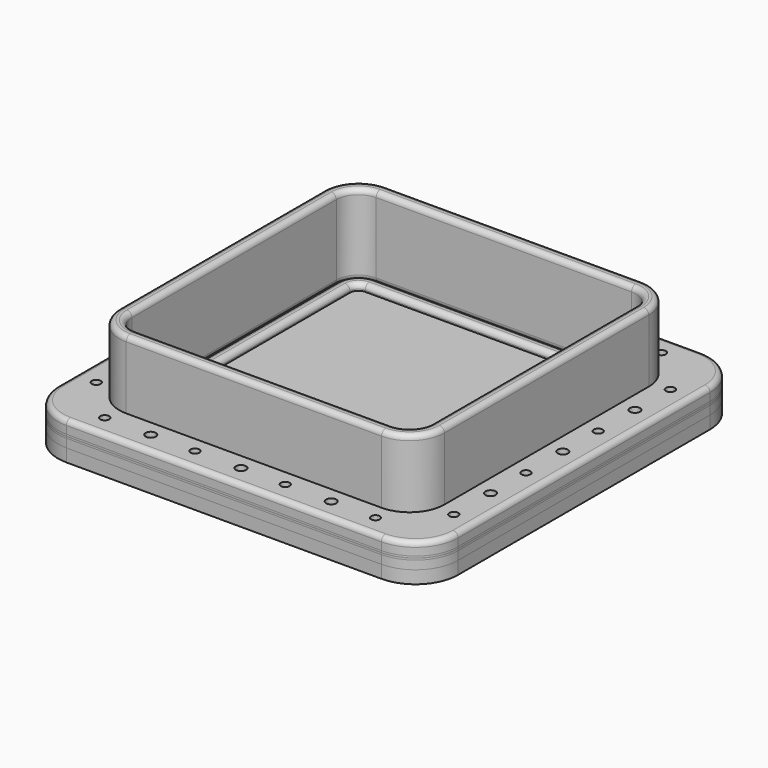
from build123d import *

# Parameters (mm, degrees)
F1_DEPTH  = 25
F2_DEPTH  = 10
F3_R      = 3
F4_DEPTH  = 7.5
F6_DEPTH  = 25
F8_DEPTH  = 40
F9_R      = 3
F10_R     = 3
F11_R     = 2.6
F13_DEPTH = 25
F14_R     = 2.6
F15_DEPTH = 1
F16_R     = 2.6
F17_DEPTH = 0.1
F18_R     = 2.6
F19_DEPTH = 1
F20_R     = 2.6
F21_DEPTH = 5
F23_DEPTH = 7.5
F25_DEPTH = 10
F26_R     = 3
F28_D     = 6
F28_2_D   = 6
F28_3_D   = 6
F28_4_D   = 6
F28_5_D   = 6
F28_6_D   = 6


# Not quite as in the source:
# - a feature names something its author has since deleted; it is built from what else it names


with BuildPart() as f1:
    # F0 (on Top) → F1 (new body)
    with BuildSketch(Plane.XY):
        with BuildLine():
            Line((-75, -87.5), (75, -87.5))
            ThreePointArc((75, -87.5), (83.8388347648, -83.8388347648), (87.5, -75))
            Line((87.5, -75), (87.5, 75))
            ThreePointArc((87.5, 75), (83.8388347648, 83.8388347648), (75, 87.5))
            Line((75, 87.5), (-75, 87.5))
            ThreePointArc((-75, 87.5), (-83.8388347648, 83.8388347648), (-87.5, 75))
            Line((-87.5, 75), (-87.5, -75))
            ThreePointArc((-87.5, -75), (-83.8388347648, -83.8388347648), (-75, -87.5))
        make_face()
        with BuildLine():
            ThreePointArc((80, -75), (78.5355339059, -78.5355339059), (75, -80))
            Line((75, -80), (-75, -80))
            ThreePointArc((-75, -80), (-78.5355339059, -78.5355339059), (-80, -75))
            Line((-80, -75), (-80, 75))
            ThreePointArc((-80, 75), (-78.5355339059, 78.5355339059), (-75, 80))
            Line((-75, 80), (75, 80))
            ThreePointArc((75, 80), (78.5355339059, 78.5355339059), (80, 75))
            Line((80, 75), (80, -75))
        make_face(mode=Mode.SUBTRACT)
    extrude(amount=F1_DEPTH)

    # F0 (on Top) → F2 (join)
    with BuildSketch(Plane.XY):
        with BuildLine():
            Line((-92.5, -117.5), (92.5, -117.5))
            ThreePointArc((92.5, -117.5), (110.1776695297, -110.1776695297), (117.5, -92.5))
            Line((117.5, -92.5), (117.5, 92.5))
            ThreePointArc((117.5, 92.5), (110.1776695297, 110.1776695297), (92.5, 117.5))
            Line((92.5, 117.5), (-92.5, 117.5))
            ThreePointArc((-92.5, 117.5), (-110.1776695297, 110.1776695297), (-117.5, 92.5))
            Line((-117.5, 92.5), (-117.5, -92.5))
            ThreePointArc((-117.5, -92.5), (-110.1776695297, -110.1776695297), (-92.5, -117.5))
        make_face()
        with BuildLine():
            ThreePointArc((87.5, -75), (83.8388347648, -83.8388347648), (75, -87.5))
            Line((75, -87.5), (-75, -87.5))
            ThreePointArc((-75, -87.5), (-83.8388347648, -83.8388347648), (-87.5, -75))
            Line((-87.5, -75), (-87.5, 75))
            ThreePointArc((-87.5, 75), (-83.8388347648, 83.8388347648), (-75, 87.5))
            Line((-75, 87.5), (75, 87.5))
            ThreePointArc((75, 87.5), (83.8388347648, 83.8388347648), (87.5, 75))
            Line((87.5, 75), (87.5, -75))
        make_face(mode=Mode.SUBTRACT)
    extrude(amount=F2_DEPTH)

    # F3
    f3_edges = [f1.edges().sort_by_distance(p)[0] for p in [
        (0, -87.5, 25),
        (83.838835, -83.838835, 25),
        (87.5, 0, 25),
        (83.838835, 83.838835, 25),
        (0, 87.5, 25),
        (-83.838835, 83.838835, 25),
        (-87.5, 0, 25),
        (-83.838835, -83.838835, 25),
        (78.535534, -78.535534, 25),
        (0, -80, 25),
        (-78.535534, -78.535534, 25),
        (-80, 0, 25),
        (-78.535534, 78.535534, 25),
        (0, 80, 25),
        (78.535534, 78.535534, 25),
        (80, 0, 25),
    ]]
    fillet(f3_edges, radius=F3_R)


with BuildPart() as f4:
    # F4 (new): a face of the model
    f4_faces = [f1.part.faces().sort_by_distance(p)[0] for p in [
        (-107.8276695297, -107.8276695297, 10),
    ]]
    extrude(f4_faces, amount=F4_DEPTH)


with BuildPart() as f6_tool:
    # F5 (on face) → F6 (new body)
    with BuildSketch(Plane.XY.offset(17.5)):
        with BuildLine():
            Line((-75, -88), (75, -88))
            ThreePointArc((75, -88), (84.1923881554, -84.1923881554), (88, -75))
            Line((88, -75), (88, 75))
            ThreePointArc((88, 75), (84.1923881554, 84.1923881554), (75, 88))
            Line((75, 88), (-75, 88))
            ThreePointArc((-75, 88), (-84.1923881554, 84.1923881554), (-88, 75))
            Line((-88, 75), (-88, -75))
            ThreePointArc((-88, -75), (-84.1923881554, -84.1923881554), (-75, -88))
        make_face()
    extrude(amount=-F6_DEPTH)


with BuildPart() as f1_1:
    add(f1.part)

    # F6: cut by f6_tool
    add(f6_tool.part, mode=Mode.SUBTRACT)


with BuildPart() as f4_1:
    add(f4.part)

    # F6: cut by f6_tool
    add(f6_tool.part, mode=Mode.SUBTRACT)

    # F7 (on face) → F8 (join)
    with BuildSketch(Plane.XY.offset(17.5)):
        with BuildLine():
            Line((-75, -95.5), (75, -95.5))
            ThreePointArc((75, -95.5), (89.4956890143, -89.4956890143), (95.5, -75))
            Line((95.5, -75), (95.5, 75))
            ThreePointArc((95.5, 75), (89.4956890143, 89.4956890143), (75, 95.5))
            Line((75, 95.5), (-75, 95.5))
            ThreePointArc((-75, 95.5), (-89.4956890143, 89.4956890143), (-95.5, 75))
            Line((-95.5, 75), (-95.5, -75))
            ThreePointArc((-95.5, -75), (-89.4956890143, -89.4956890143), (-75, -95.5))
        make_face()
        with BuildLine():
            ThreePointArc((88, -75), (84.1923881554, -84.1923881554), (75, -88))
            Line((75, -88), (-75, -88))
            ThreePointArc((-75, -88), (-84.1923881554, -84.1923881554), (-88, -75))
            Line((-88, -75), (-88, 75))
            ThreePointArc((-88, 75), (-84.1923881554, 84.1923881554), (-75, 88))
            Line((-75, 88), (75, 88))
            ThreePointArc((75, 88), (84.1923881554, 84.1923881554), (88, 75))
            Line((88, 75), (88, -75))
        make_face(mode=Mode.SUBTRACT)
    extrude(amount=F8_DEPTH)

    # F9
    f9_edges = [f4_1.edges().sort_by_distance(p)[0] for p in [
        (0, -95.5, 57.5),
        (89.495689, -89.495689, 57.5),
        (95.5, 0, 57.5),
        (89.495689, 89.495689, 57.5),
        (0, 95.5, 57.5),
        (-89.495689, 89.495689, 57.5),
        (-95.5, 0, 57.5),
        (-89.495689, -89.495689, 57.5),
        (84.192388, -84.192388, 57.5),
        (0, -88, 57.5),
        (-84.192388, -84.192388, 57.5),
        (-88, 0, 57.5),
        (-84.192388, 84.192388, 57.5),
        (0, 88, 57.5),
        (84.192388, 84.192388, 57.5),
        (88, 0, 57.5),
        (0, 117.5, 17.5),
    ]]
    fillet(f9_edges, radius=F9_R)

    # F10
    f10_edges = [f4_1.edges().sort_by_distance(p)[0] for p in [
        (0, -88, 10),
    ]]
    fillet(f10_edges, radius=F10_R)

    # F11 (on face) → F13 (cut)
    with BuildSketch(Plane(origin=(0, 0, 0), x_dir=(1, 0, 0), z_dir=(0, 0, -1))):
        with Locations((-80, 105)):
            Circle(F11_R)
        with Locations((-105, 80)):
            Circle(F11_R)
        with Locations((-80, -105)):
            Circle(F11_R)
        with Locations((-27, 105)):
            Circle(F11_R)
        with Locations((-27, -105)):
            Circle(F11_R)
        with Locations((26, 105)):
            Circle(F11_R)
        with Locations((26, -105)):
            Circle(F11_R)
        with Locations((79, 105)):
            Circle(F11_R)
        with Locations((79, -105)):
            Circle(F11_R)
        with Locations((-105, 27)):
            Circle(F11_R)
        with Locations((-105, -26)):
            Circle(F11_R)
        with Locations((-105, -79)):
            Circle(F11_R)
        with Locations((105, 80)):
            Circle(F11_R)
        with Locations((105, 27)):
            Circle(F11_R)
        with Locations((105, -26)):
            Circle(F11_R)
        with Locations((105, -79)):
            Circle(F11_R)
    extrude(amount=-F13_DEPTH, mode=Mode.SUBTRACT)

    # F28 (through all)
    with Locations(Plane(origin=(0, 0, -4.6), x_dir=(1, 0, 0), z_dir=(0, 0, -1))):
        with Locations((-105, 53), (-105, 0), (-105, -53), (-53, -105), (0, -105), (53, -105), (105, -53), (105, 0), (105, 53), (53, 105), (0, 105), (-53, 105)):
            Hole(F28_D / 2)


with BuildPart() as f15:
    # F14 (on face) → F15 (new body)
    with BuildSketch(Plane(origin=(0, 0, 10), x_dir=(1, 0, 0), z_dir=(0, 0, -1))):
        with BuildLine():
            ThreePointArc((117.5, 92.5), (110.1776695297, 110.1776695297), (92.5, 117.5))
            Line((92.5, 117.5), (-92.5, 117.5))
            ThreePointArc((-92.5, 117.5), (-110.1776695297, 110.1776695297), (-117.5, 92.5))
            Line((-117.5, 92.5), (-117.5, -92.5))
            ThreePointArc((-117.5, -92.5), (-110.1776695297, -110.1776695297), (-92.5, -117.5))
            Line((-92.5, -117.5), (92.5, -117.5))
            ThreePointArc((92.5, -117.5), (110.1776695297, -110.1776695297), (117.5, -92.5))
            Line((117.5, -92.5), (117.5, 92.5))
        make_face()
        with Locations((-80, -105)):
            Circle(F14_R, mode=Mode.SUBTRACT)
        with Locations((-105, -79)):
            Circle(F14_R, mode=Mode.SUBTRACT)
        with Locations((-27, -105)):
            Circle(F14_R, mode=Mode.SUBTRACT)
        with Locations((-105, -26)):
            Circle(F14_R, mode=Mode.SUBTRACT)
        with Locations((26, -105)):
            Circle(F14_R, mode=Mode.SUBTRACT)
        with Locations((79, -105)):
            Circle(F14_R, mode=Mode.SUBTRACT)
        with Locations((105, -79)):
            Circle(F14_R, mode=Mode.SUBTRACT)
        with Locations((105, -26)):
            Circle(F14_R, mode=Mode.SUBTRACT)
        with Locations((-105, 27)):
            Circle(F14_R, mode=Mode.SUBTRACT)
        with Locations((-105, 80)):
            Circle(F14_R, mode=Mode.SUBTRACT)
        with Locations((-80, 105)):
            Circle(F14_R, mode=Mode.SUBTRACT)
        with Locations((-27, 105)):
            Circle(F14_R, mode=Mode.SUBTRACT)
        with BuildLine():
            ThreePointArc((91, -75), (86.313708499, -86.313708499), (75, -91))
            Line((75, -91), (-75, -91))
            ThreePointArc((-75, -91), (-86.313708499, -86.313708499), (-91, -75))
            Line((-91, -75), (-91, 75))
            ThreePointArc((-91, 75), (-86.313708499, 86.313708499), (-75, 91))
            Line((-75, 91), (75, 91))
            ThreePointArc((75, 91), (86.313708499, 86.313708499), (91, 75))
            Line((91, 75), (91, -75))
        make_face(mode=Mode.SUBTRACT)
        with Locations((105, 27)):
            Circle(F14_R, mode=Mode.SUBTRACT)
        with Locations((26, 105)):
            Circle(F14_R, mode=Mode.SUBTRACT)
        with Locations((105, 80)):
            Circle(F14_R, mode=Mode.SUBTRACT)
        with Locations((79, 105)):
            Circle(F14_R, mode=Mode.SUBTRACT)
    extrude(amount=F15_DEPTH)

    # F28#2 (through all)
    with Locations(Plane(origin=(0, 0, -4.6), x_dir=(1, 0, 0), z_dir=(0, 0, -1))):
        with Locations((-105, 53), (-105, 0), (-105, -53), (-53, -105), (0, -105), (53, -105), (105, -53), (105, 0), (105, 53), (53, 105), (0, 105), (-53, 105)):
            Hole(F28_2_D / 2)


with BuildPart() as f17:
    # F16 (on face) → F17 (new body)
    with BuildSketch(Plane(origin=(0, 0, 9), x_dir=(1, 0, 0), z_dir=(0, 0, -1))):
        with BuildLine():
            ThreePointArc((117.5, 92.5), (110.1776695297, 110.1776695297), (92.5, 117.5))
            Line((92.5, 117.5), (-92.5, 117.5))
            ThreePointArc((-92.5, 117.5), (-110.1776695297, 110.1776695297), (-117.5, 92.5))
            Line((-117.5, 92.5), (-117.5, -92.5))
            ThreePointArc((-117.5, -92.5), (-110.1776695297, -110.1776695297), (-92.5, -117.5))
            Line((-92.5, -117.5), (92.5, -117.5))
            ThreePointArc((92.5, -117.5), (110.1776695297, -110.1776695297), (117.5, -92.5))
            Line((117.5, -92.5), (117.5, 92.5))
        make_face()
        with Locations((-80, -105)):
            Circle(F16_R, mode=Mode.SUBTRACT)
        with Locations((-105, -79)):
            Circle(F16_R, mode=Mode.SUBTRACT)
        with Locations((-27, -105)):
            Circle(F16_R, mode=Mode.SUBTRACT)
        with Locations((-105, -26)):
            Circle(F16_R, mode=Mode.SUBTRACT)
        with Locations((26, -105)):
            Circle(F16_R, mode=Mode.SUBTRACT)
        with Locations((79, -105)):
            Circle(F16_R, mode=Mode.SUBTRACT)
        with Locations((105, -79)):
            Circle(F16_R, mode=Mode.SUBTRACT)
        with Locations((105, -26)):
            Circle(F16_R, mode=Mode.SUBTRACT)
        with Locations((-105, 27)):
            Circle(F16_R, mode=Mode.SUBTRACT)
        with Locations((-105, 80)):
            Circle(F16_R, mode=Mode.SUBTRACT)
        with Locations((-80, 105)):
            Circle(F16_R, mode=Mode.SUBTRACT)
        with Locations((-27, 105)):
            Circle(F16_R, mode=Mode.SUBTRACT)
        with Locations((105, 27)):
            Circle(F16_R, mode=Mode.SUBTRACT)
        with Locations((26, 105)):
            Circle(F16_R, mode=Mode.SUBTRACT)
        with Locations((105, 80)):
            Circle(F16_R, mode=Mode.SUBTRACT)
        with Locations((79, 105)):
            Circle(F16_R, mode=Mode.SUBTRACT)
    extrude(amount=F17_DEPTH)

    # F28#3 (through all)
    with Locations(Plane(origin=(0, 0, -4.6), x_dir=(1, 0, 0), z_dir=(0, 0, -1))):
        with Locations((-105, 53), (-105, 0), (-105, -53), (-53, -105), (0, -105), (53, -105), (105, -53), (105, 0), (105, 53), (53, 105), (0, 105), (-53, 105)):
            Hole(F28_3_D / 2)


with BuildPart() as f19:
    # F18 (on face) → F19 (new body)
    with BuildSketch(Plane(origin=(0, 0, 8.9), x_dir=(1, 0, 0), z_dir=(0, 0, -1))):
        with BuildLine():
            ThreePointArc((117.5, 92.5), (110.1776695297, 110.1776695297), (92.5, 117.5))
            Line((92.5, 117.5), (-92.5, 117.5))
            ThreePointArc((-92.5, 117.5), (-110.1776695297, 110.1776695297), (-117.5, 92.5))
            Line((-117.5, 92.5), (-117.5, -92.5))
            ThreePointArc((-117.5, -92.5), (-110.1776695297, -110.1776695297), (-92.5, -117.5))
            Line((-92.5, -117.5), (92.5, -117.5))
            ThreePointArc((92.5, -117.5), (110.1776695297, -110.1776695297), (117.5, -92.5))
            Line((117.5, -92.5), (117.5, 92.5))
        make_face()
        with Locations((-80, -105)):
            Circle(F18_R, mode=Mode.SUBTRACT)
        with Locations((-105, -79)):
            Circle(F18_R, mode=Mode.SUBTRACT)
        with Locations((-27, -105)):
            Circle(F18_R, mode=Mode.SUBTRACT)
        with Locations((-105, -26)):
            Circle(F18_R, mode=Mode.SUBTRACT)
        with Locations((26, -105)):
            Circle(F18_R, mode=Mode.SUBTRACT)
        with Locations((79, -105)):
            Circle(F18_R, mode=Mode.SUBTRACT)
        with Locations((105, -79)):
            Circle(F18_R, mode=Mode.SUBTRACT)
        with Locations((105, -26)):
            Circle(F18_R, mode=Mode.SUBTRACT)
        with Locations((-105, 27)):
            Circle(F18_R, mode=Mode.SUBTRACT)
        with Locations((-105, 80)):
            Circle(F18_R, mode=Mode.SUBTRACT)
        with Locations((-80, 105)):
            Circle(F18_R, mode=Mode.SUBTRACT)
        with Locations((-27, 105)):
            Circle(F18_R, mode=Mode.SUBTRACT)
        with BuildLine():
            ThreePointArc((-91, 75), (-86.313708499, 86.313708499), (-75, 91))
            Line((-75, 91), (75, 91))
            ThreePointArc((75, 91), (86.313708499, 86.313708499), (91, 75))
            Line((91, 75), (91, -75))
            ThreePointArc((91, -75), (86.313708499, -86.313708499), (75, -91))
            Line((75, -91), (-75, -91))
            ThreePointArc((-75, -91), (-86.313708499, -86.313708499), (-91, -75))
            Line((-91, -75), (-91, 75))
        make_face(mode=Mode.SUBTRACT)
        with Locations((105, 27)):
            Circle(F18_R, mode=Mode.SUBTRACT)
        with Locations((26, 105)):
            Circle(F18_R, mode=Mode.SUBTRACT)
        with Locations((105, 80)):
            Circle(F18_R, mode=Mode.SUBTRACT)
        with Locations((79, 105)):
            Circle(F18_R, mode=Mode.SUBTRACT)
    extrude(amount=F19_DEPTH)

    # F28#4 (through all)
    with Locations(Plane(origin=(0, 0, -4.6), x_dir=(1, 0, 0), z_dir=(0, 0, -1))):
        with Locations((-105, 53), (-105, 0), (-105, -53), (-53, -105), (0, -105), (53, -105), (105, -53), (105, 0), (105, 53), (53, 105), (0, 105), (-53, 105)):
            Hole(F28_4_D / 2)


with BuildPart() as f21:
    # F20 (on face) → F21 (new body)
    with BuildSketch(Plane(origin=(0, 0, 7.9), x_dir=(1, 0, 0), z_dir=(0, 0, -1))):
        with BuildLine():
            ThreePointArc((117.5, 92.5), (110.1776695297, 110.1776695297), (92.5, 117.5))
            Line((92.5, 117.5), (-92.5, 117.5))
            ThreePointArc((-92.5, 117.5), (-110.1776695297, 110.1776695297), (-117.5, 92.5))
            Line((-117.5, 92.5), (-117.5, -92.5))
            ThreePointArc((-117.5, -92.5), (-110.1776695297, -110.1776695297), (-92.5, -117.5))
            Line((-92.5, -117.5), (92.5, -117.5))
            ThreePointArc((92.5, -117.5), (110.1776695297, -110.1776695297), (117.5, -92.5))
            Line((117.5, -92.5), (117.5, 92.5))
        make_face()
        with Locations((-80, -105)):
            Circle(F20_R, mode=Mode.SUBTRACT)
        with Locations((-105, -79)):
            Circle(F20_R, mode=Mode.SUBTRACT)
        with Locations((-27, -105)):
            Circle(F20_R, mode=Mode.SUBTRACT)
        with Locations((-105, -26)):
            Circle(F20_R, mode=Mode.SUBTRACT)
        with Locations((26, -105)):
            Circle(F20_R, mode=Mode.SUBTRACT)
        with Locations((79, -105)):
            Circle(F20_R, mode=Mode.SUBTRACT)
        with Locations((105, -79)):
            Circle(F20_R, mode=Mode.SUBTRACT)
        with Locations((105, -26)):
            Circle(F20_R, mode=Mode.SUBTRACT)
        with Locations((-105, 27)):
            Circle(F20_R, mode=Mode.SUBTRACT)
        with Locations((-105, 80)):
            Circle(F20_R, mode=Mode.SUBTRACT)
        with Locations((-80, 105)):
            Circle(F20_R, mode=Mode.SUBTRACT)
        with Locations((-27, 105)):
            Circle(F20_R, mode=Mode.SUBTRACT)
        with BuildLine():
            Line((-91, -75), (-91, 75))
            ThreePointArc((-91, 75), (-86.313708499, 86.313708499), (-75, 91))
            Line((-75, 91), (75, 91))
            ThreePointArc((75, 91), (86.313708499, 86.313708499), (91, 75))
            Line((91, 75), (91, -75))
            ThreePointArc((91, -75), (86.313708499, -86.313708499), (75, -91))
            Line((75, -91), (-75, -91))
            ThreePointArc((-75, -91), (-86.313708499, -86.313708499), (-91, -75))
        make_face(mode=Mode.SUBTRACT)
        with Locations((105, 27)):
            Circle(F20_R, mode=Mode.SUBTRACT)
        with Locations((26, 105)):
            Circle(F20_R, mode=Mode.SUBTRACT)
        with Locations((105, 80)):
            Circle(F20_R, mode=Mode.SUBTRACT)
        with Locations((79, 105)):
            Circle(F20_R, mode=Mode.SUBTRACT)
    extrude(amount=F21_DEPTH)

    # F28#5 (through all)
    with Locations(Plane(origin=(0, 0, -4.6), x_dir=(1, 0, 0), z_dir=(0, 0, -1))):
        with Locations((-105, 53), (-105, 0), (-105, -53), (-53, -105), (0, -105), (53, -105), (105, -53), (105, 0), (105, 53), (53, 105), (0, 105), (-53, 105)):
            Hole(F28_5_D / 2)


with BuildPart() as f23:
    # F22 (on face) → F23 (new body)
    with BuildSketch(Plane(origin=(0, 0, 2.9), x_dir=(1, 0, 0), z_dir=(0, 0, -1))):
        with BuildLine():
            ThreePointArc((117.5, 92.5), (110.1776695297, 110.1776695297), (92.5, 117.5))
            Line((92.5, 117.5), (-92.5, 117.5))
            ThreePointArc((-92.5, 117.5), (-110.1776695297, 110.1776695297), (-117.5, 92.5))
            Line((-117.5, 92.5), (-117.5, -92.5))
            ThreePointArc((-117.5, -92.5), (-110.1776695297, -110.1776695297), (-92.5, -117.5))
            Line((-92.5, -117.5), (92.5, -117.5))
            ThreePointArc((92.5, -117.5), (110.1776695297, -110.1776695297), (117.5, -92.5))
            Line((117.5, -92.5), (117.5, 92.5))
        make_face()
        with BuildLine():
            Line((-75, 87.5), (75, 87.5))
            ThreePointArc((75, 87.5), (83.8388347648, 83.8388347648), (87.5, 75))
            Line((87.5, 75), (87.5, -75))
            ThreePointArc((87.5, -75), (83.8388347648, -83.8388347648), (75, -87.5))
            Line((75, -87.5), (-75, -87.5))
            ThreePointArc((-75, -87.5), (-83.8388347648, -83.8388347648), (-87.5, -75))
            Line((-87.5, -75), (-87.5, 75))
            ThreePointArc((-87.5, 75), (-83.8388347648, 83.8388347648), (-75, 87.5))
        make_face(mode=Mode.SUBTRACT)
        with BuildLine():
            ThreePointArc((87.5, 75), (83.8388347648, 83.8388347648), (75, 87.5))
            Line((75, 87.5), (-75, 87.5))
            ThreePointArc((-75, 87.5), (-83.8388347648, 83.8388347648), (-87.5, 75))
            Line((-87.5, 75), (-87.5, -75))
            ThreePointArc((-87.5, -75), (-83.8388347648, -83.8388347648), (-75, -87.5))
            Line((-75, -87.5), (75, -87.5))
            ThreePointArc((75, -87.5), (83.8388347648, -83.8388347648), (87.5, -75))
            Line((87.5, -75), (87.5, 75))
        make_face()
        with BuildLine():
            Line((-75, 80), (75, 80))
            ThreePointArc((75, 80), (78.5355339059, 78.5355339059), (80, 75))
            Line((80, 75), (80, -75))
            ThreePointArc((80, -75), (78.5355339059, -78.5355339059), (75, -80))
            Line((75, -80), (-75, -80))
            ThreePointArc((-75, -80), (-78.5355339059, -78.5355339059), (-80, -75))
            Line((-80, -75), (-80, 75))
            ThreePointArc((-80, 75), (-78.5355339059, 78.5355339059), (-75, 80))
        make_face(mode=Mode.SUBTRACT)
    extrude(amount=F23_DEPTH)

    # F24 (on face) → F25 (join)
    with BuildSketch(Plane.XY.offset(2.9)):
        with BuildLine():
            ThreePointArc((87.5, 75), (83.8388347648, 83.8388347648), (75, 87.5))
            Line((75, 87.5), (-75, 87.5))
            ThreePointArc((-75, 87.5), (-83.8388347648, 83.8388347648), (-87.5, 75))
            Line((-87.5, 75), (-87.5, -75))
            ThreePointArc((-87.5, -75), (-83.8388347648, -83.8388347648), (-75, -87.5))
            Line((-75, -87.5), (75, -87.5))
            ThreePointArc((75, -87.5), (83.8388347648, -83.8388347648), (87.5, -75))
            Line((87.5, -75), (87.5, 75))
        make_face()
        with BuildLine():
            ThreePointArc((80, -75), (78.5355339059, -78.5355339059), (75, -80))
            Line((75, -80), (-75, -80))
            ThreePointArc((-75, -80), (-78.5355339059, -78.5355339059), (-80, -75))
            Line((-80, -75), (-80, 75))
            ThreePointArc((-80, 75), (-78.5355339059, 78.5355339059), (-75, 80))
            Line((-75, 80), (75, 80))
            ThreePointArc((75, 80), (78.5355339059, 78.5355339059), (80, 75))
            Line((80, 75), (80, -75))
        make_face(mode=Mode.SUBTRACT)
    extrude(amount=F25_DEPTH)

    # F26
    f26_edges = [f23.edges().sort_by_distance(p)[0] for p in [
        (83.838835, 83.838835, 12.9),
        (0, 87.5, 12.9),
        (-83.838835, 83.838835, 12.9),
        (-87.5, 0, 12.9),
        (-83.838835, -83.838835, 12.9),
        (0, -87.5, 12.9),
        (83.838835, -83.838835, 12.9),
        (87.5, 0, 12.9),
        (78.535534, -78.535534, 12.9),
        (0, -80, 12.9),
        (-78.535534, -78.535534, 12.9),
        (-80, 0, 12.9),
        (-78.535534, 78.535534, 12.9),
        (0, 80, 12.9),
        (78.535534, 78.535534, 12.9),
        (80, 0, 12.9),
    ]]
    fillet(f26_edges, radius=F26_R)

    # F28#6 (through all)
    with Locations(Plane(origin=(0, 0, -4.6), x_dir=(1, 0, 0), z_dir=(0, 0, -1))):
        with Locations((-105, 53), (-105, 0), (-105, -53), (-53, -105), (0, -105), (53, -105), (105, -53), (105, 0), (105, 53), (53, 105), (0, 105), (-53, 105)):
            Hole(F28_6_D / 2)


solid = Compound([f4_1.part, f15.part, f17.part, f19.part, f21.part, f23.part])
